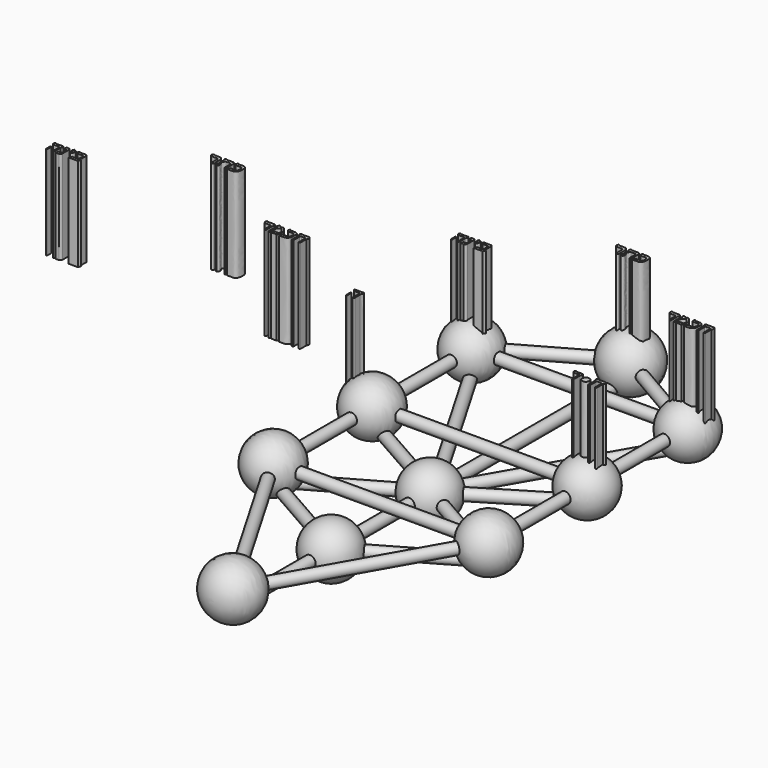
from build123d import *

# Parameters (mm, degrees)
F25_W     = 57.1091186851
F25_H     = 1.5
F25_W_2   = 52.1633550525
F38_DEPTH = 25


# Not quite as in the source:
# - ends of sketch curves that miss each other by under 0.0002 mm in the source are joined


with BuildPart() as f1:
    # F0 (on Top) → F1 (revolve)
    with BuildSketch(Plane.XY):
        with BuildLine():
            Line((-29.2246792197, -9.2726029596), (-29.2246792197, -23.7725834981))
            ThreePointArc((-29.2246792197, -23.7725834981), (-21.9628008624, -16.5225932289), (-29.2246792197, -9.2726029596))
        make_face()
    revolve(axis=Axis((-29.2246792197, -16.5225932289, 0), (0, -1, 0)))


with BuildPart() as f2:
    # F0 (on Top) → F2 (revolve)
    with BuildSketch(Plane.XY):
        with BuildLine():
            Line((28.2959174365, -23.6783408071), (28.2959174365, -9.1783614346))
            ThreePointArc((28.2959174365, -9.1783614346), (21.0581464556, -16.4283511208), (28.2959174365, -23.6783408071))
        make_face()
    revolve(axis=Axis((28.2959174365, -16.4283511208, 0), (0, -1, 0)))


with BuildPart() as f3:
    # F0 (on Top) → F3 (revolve)
    with BuildSketch(Plane.XY):
        with BuildLine():
            Line((-29.1159380303, 23.6979271757), (-29.254943913, 9.1995414743))
            ThreePointArc((-29.254943913, 9.1995414743), (-21.8528783148, 16.3784320606), (-29.1159380303, 23.6979271757))
        make_face()
    revolve(axis=Axis((-29.1854409717, 16.448734325, 0), (-0.0095872394, -0.9999540414, 0)))


with BuildPart() as f4:
    # F0 (on Top) → F4 (revolve)
    with BuildSketch(Plane.XY):
        with BuildLine():
            Line((-29.1507775773, 57.0575961277), (-29.1507775773, 42.5576208684))
            ThreePointArc((-29.1507775773, 42.5576208684), (-21.9141704929, 49.807608498), (-29.1507775773, 57.0575961277))
        make_face()
    revolve(axis=Axis((-29.1507775773, 49.807608498, 0), (0, 1, 0)))


with BuildPart() as f5:
    # F0 (on Top) → F5 (revolve)
    with BuildSketch(Plane.XY):
        with BuildLine():
            Line((-0.3091844796, -58.8778027446), (-0.3091844796, -73.3646112209))
            ThreePointArc((-0.3091844796, -73.3646112209), (7.25, -66.1212069828), (-0.3091844796, -58.8778027446))
        make_face()
    revolve(axis=Axis((-0.3091844796, -66.1212069828, 0), (0, -1, 0)))


with BuildPart() as f6:
    # F0 (on Top) → F6 (revolve)
    with BuildSketch(Plane.XY):
        with BuildLine():
            Line((35.5459174365, 16.4479395461), (21.0459174365, 16.4479395461))
            ThreePointArc((21.0459174365, 16.4479395461), (28.2959174365, 9.1979395461), (35.5459174365, 16.4479395461))
        make_face()
    revolve(axis=Axis((28.2959174365, 16.4479395461, 0), (1, 0, 0)))


with BuildPart() as f7:
    # F0 (on Top) → F7 (revolve)
    with BuildSketch(Plane.XY):
        with BuildLine():
            Line((28.5925234624, 42.4439817941), (28.5925234624, 56.9430380786))
            ThreePointArc((28.5925234624, 56.9430380786), (21.4252381199, 49.6935099363), (28.5925234624, 42.4439817941))
        make_face()
    revolve(axis=Axis((28.5925234624, 49.6935099363, 0), (0, 1, 0)))


with BuildPart() as f8:
    # F0 (on Top) → F8 (revolve)
    with BuildSketch(Plane.XY):
        with BuildLine():
            Line((0, 58.9001502285), (0, 66.3991495967))
            Line((0, 66.3991495967), (0, 73.7951572397))
            ThreePointArc((0, 73.7951572397), (-7.7135701863, 66.3476537341), (0, 58.9001502285))
        make_face()
    revolve(axis=Axis((0, 66.3476537341, 0), (0, -1, 0)))


with BuildPart() as f11:
    # F10 (on offset) → F11 (revolve)
    with BuildSketch(Plane.XY.offset(-4.1)):
        with BuildLine():
            ThreePointArc((-0.4545195449, -40.3316861829), (6.7954804551, -33.0816861829), (-0.4545195449, -25.8316861829))
            Line((-0.4545195449, -25.8316861829), (-0.4545195449, -40.3316861829))
        make_face()
    revolve(axis=Axis((-0.4545195449, -33.0816861829, -4.1), (0, -1, 0)))


with BuildPart() as f11b:
    # F10 (on offset) → F11, piece 2 (revolve)
    with BuildSketch(Plane.XY.offset(-4.1)):
        with BuildLine():
            Line((-0.4545195449, 0), (-0.4545195449, -7.25))
            ThreePointArc((-0.4545195449, -7.25), (6.7954804551, 0), (-0.4545195449, 7.25))
            Line((-0.4545195449, 7.25), (-0.4545195449, 0))
        make_face()
    revolve(axis=Axis((-0.4545195449, -33.0816861829, -4.1), (0, -1, 0)))


with BuildPart() as f13:
    # F12 (on offset) → F13 (revolve)
    with BuildSketch(Plane.XY.offset(-4.1)):
        Polygon((-26.0090909671, -16.1936523754), (-5.0356983319, -4.2643418488), (-1.3323071181, -2.1579156468), (-1.9716815625, -0.7959197113), (-5.7773049848, -2.9604938621), (-27.1052462657, -15.0914656538), align=None)
    revolve(axis=Axis((-16.4412756253, -9.025979758, -4.1), (-0.8692319911, -0.4944044353, 0)))


with BuildPart() as f14:
    # F12 (on offset) → F14 (revolve)
    with BuildSketch(Plane.XY.offset(-4.1)):
        Polygon((-1.129006822, 1.2827262948), (-0.3514380131, 0), (5.1909224811, 3.3596930733), (23.0870766217, 14.2080644789), (27.8991724979, 17.1250824535), (27.1465061848, 18.4229042555), (20.3817308309, 14.322202231), (4.3483456761, 4.603012528), align=None)
    revolve(axis=Axis((14.1389995514, 8.7838787761, -4.1), (0.8551508632, 0.5183792059, 0)))


with BuildPart() as f15:
    # F12 (on offset) → F15 (revolve)
    with BuildSketch(Plane.XY.offset(-4.1)):
        Polygon((-28.9924826053, 15.1554377692), (-25.2247012465, 13.0175819941), (-7.1870962072, 2.7829652716), (-2.8568617599, 0), (-1.9319412235, 1.525806948), (-6.4468489258, 4.0875855085), (-24.4844539652, 14.322202231), (-28.0564903249, 16.3489914295), align=None)
    revolve(axis=Axis((-15.4656514455, 9.2048938697, -4.1), (-0.8697468246, 0.4934981876, 0)))


with BuildPart() as f16:
    # F12 (on offset) → F16 (revolve)
    with BuildSketch(Plane.XY.offset(-4.1)):
        Polygon((3.2083909627, -1.937990184), (2.4637627258, -3.2401149049), (25.1154975479, -16.1936523754), (25.8601257848, -14.8915276545), align=None)
    revolve(axis=Axis((14.5342583738, -8.4147589193, -4.1), (0.8680831473, -0.4964188246, 0)))


with BuildPart() as f17:
    # F12 (on offset) → F17 (revolve)
    with BuildSketch(Plane.XY.offset(-4.1)):
        Polygon((-0.2782110823, 62.3477734625), (-1.7782110823, 62.4405108392), (-1.7782110823, 3.2196498942), (-0.2782110823, 3.2196498942), align=None)
    revolve(axis=Axis((-0.2782110823, 32.7837116783, -4.1), (0, -1, 0)))


with BuildPart() as f18:
    # F12 (on offset) → F18 (revolve)
    with BuildSketch(Plane.XY.offset(-4.1)):
        Polygon((-26.5824754433, -18.0288977431), (-27.3254525627, -19.3319652778), (-6.591141076, -31.1541606829), (-3.0596121292, -33.1677517932), (-2.3166350098, -31.8646842584), (-5.8412572049, -29.8550312084), align=None)
    revolve(axis=Axis((-16.2118663241, -23.9419644758, -4.1), (-0.8687116898, 0.4953180796, 0)))


with BuildPart() as f19:
    # F12 (on offset) → F19 (revolve)
    with BuildSketch(Plane.XY.offset(-4.1)):
        Polygon((1.202256309, -32.0779555323), (1.8714931815, -33.4234479594), (26.3763282511, -19.3291654157), (25.6284619664, -18.0288977431), align=None)
    revolve(axis=Axis((13.4153591377, -25.0534266377, -4.1), (-0.866845115, -0.4985775231, 0)))


with BuildPart() as f20:
    # F12 (on offset) → F20 (revolve)
    with BuildSketch(Plane.XY.offset(-4.1)):
        Polygon((-1.9146180712, -4.3942993507), (-1.9146180712, -26.9383080304), (-1.9146180712, -32.1800261736), (-0.4146180712, -32.1359224617), (-0.4146180712, -26.8926918507), (-0.4146180712, -4.3942993507), align=None)
    revolve(axis=Axis((-0.4146180712, -15.6434956007, -4.1), (0, -1, 0)))


with BuildPart() as f21:
    # F12 (on offset) → F21 (revolve)
    with BuildSketch(Plane.XY.offset(-4.1)):
        Polygon((-1.9687591121, -36.1691971211), (-1.9687591121, -62.2125818569), (-0.4687591121, -61.7515771825), (-0.4687591121, -37.240925887), align=None)
    revolve(axis=Axis((-0.4687591121, -49.4962515347, -4.1), (0, -1, 0)))


with BuildPart() as f23:
    # F22 (on offset) → F23 (revolve)
    with BuildSketch(Plane.XY.offset(-4.1)):
        Polygon((-28.4231418203, 49.4134207024), (-29.6505219667, 48.5401466053), (-0.8530344227, -0.9951512348), (0.4437502928, -0.2412617192), align=None)
    revolve(axis=Axis((-13.9896957638, 24.5860794916, -4.1), (-0.5025930104, 0.8645231437, 0)))


with BuildPart() as f24:
    # F22 (on offset) → F24 (revolve)
    with BuildSketch(Plane.XY.offset(-4.1)):
        Polygon((1.2984194251, 0.5149673192), (27.8307806202, 46.3830051455), (26.6649877391, 47.3633549421), (0, 1.266037886), align=None)
    revolve(axis=Axis((13.3324938695, 24.314696414, -4.1), (0.5007137112, 0.8656129501, 0)))


with BuildPart() as f26:
    # F25 (on Top) → F26 (revolve)
    with BuildSketch(Plane.XY):
        Polygon((-2.2483841008, 67.0031690276), (-27.4323771774, 52.753087862), (-26.6936765174, 51.4475912764), (-1.5096834408, 65.697672442), align=None)
    revolve(axis=Axis((-14.1016799791, 58.5726318592, 0), (0.8703310571, 0.4924671066, 0)))


with BuildPart() as f27:
    # F25 (on Top) → F27 (revolve)
    with BuildSketch(Plane.XY):
        Polygon((24.2450092439, 51.9837853236), (24.9992646277, 53.2803572714), (4.7837163632, 65.0403572773), (3.7131184762, 63.9278113964), align=None)
    revolve(axis=Axis((13.9790638601, 57.95579836, 0), (-0.8643812986, 0.5028369225, 0)))


with BuildPart() as f28:
    # F25 (on Top) → F28 (revolve)
    with BuildSketch(Plane.XY):
        with Locations((-0.4721774086, 49.1002261341)):
            Rectangle(F25_W, F25_H)
    revolve(axis=Axis((-0.4721774086, 49.8502261341, 0), (-1, 0, 0)))


with BuildPart() as f29:
    # F25 (on Top) → F29 (revolve)
    with BuildSketch(Plane.XY):
        with Locations((-0.4721774086, 16.0002366511)):
            Rectangle(F25_W, F25_H)
    revolve(axis=Axis((-0.4721774086, 16.7502366511, 0), (1, 0, 0)))


with BuildPart() as f30:
    # F25 (on Top) → F30 (revolve)
    with BuildSketch(Plane.XY):
        with Locations((-0.9874179959, -17.2000393569)):
            Rectangle(F25_W_2, F25_H)
    revolve(axis=Axis((-0.9874179959, -16.4500393569, 0), (1, 0, 0)))


with BuildPart() as f31:
    # F25 (on Top) → F31 (revolve)
    with BuildSketch(Plane.XY):
        Polygon((-30.5267367512, 47.590128925), (-30.5267367512, 16.7502366511), (-29.0267367512, 16.7502366511), (-29.0267367512, 47.590128925), (-29.0267367512, 48.3502261341), (-29.0267367512, 49.8502261341), (-29.0267367512, 55.475987494), (-30.5267367512, 55.475987494), align=None)
    revolve(axis=Axis((-29.0267367512, 15.1780908165, 0), (0, -1, 0)))


with BuildPart() as f32:
    # F25 (on Top) → F32 (revolve)
    with BuildSketch(Plane.XY):
        Polygon((-30.5267367512, 15.2502366511), (-30.5267367512, -17.0896556228), (-29.0267367512, -17.233947292), (-29.0267367512, -16.4500393569), (-29.0267367512, 15.2502366511), align=None)
    revolve(axis=Axis((-29.0267367512, 15.1780908165, 0), (0, -1, 0)))


with BuildPart() as f33:
    # F25 (on Top) → F33 (revolve)
    with BuildSketch(Plane.XY):
        Polygon((28.0823819339, 47.590128925), (28.0823819339, 16.7502366511), (29.5823819339, 16.7502366511), (29.5823819339, 47.590128925), (29.5823819339, 53.9458170533), (28.0823819339, 53.9458170533), (28.0823819339, 49.8502261341), (28.0823819339, 48.3502261341), align=None)
    revolve(axis=Axis((28.0823819339, 15.1531686244, 0), (0, -1, 0)))


with BuildPart() as f34:
    # F25 (on Top) → F34 (revolve)
    with BuildSketch(Plane.XY):
        Polygon((29.5823819339, 15.2502366511), (28.0823819339, 15.2502366511), (28.0823819339, -17.2837916762), (29.5823819339, -17.0896556228), align=None)
    revolve(axis=Axis((28.0823819339, 15.1531686244, 0), (0, -1, 0)))


with BuildPart() as f35:
    # F25 (on Top) → F35 (revolve)
    with BuildSketch(Plane.XY):
        Polygon((-28.1386089989, -18.5248188859), (-29.4354074421, -19.2786847874), (-3.025480399, -64.7089824118), (-2.2920486471, -62.9860143837), align=None)
    revolve(axis=Axis((-15.215328823, -40.7554166348, 0), (0.5025772677, -0.8645322955, 0)))


with BuildPart() as f36:
    # F25 (on Top) → F36 (revolve)
    with BuildSketch(Plane.XY):
        Polygon((25.1791188454, -18.5248188859), (0, -62.7821208306), (1.3037680308, -63.5238680396), (26.4828868762, -19.2665660948), align=None)
    revolve(axis=Axis((13.8933274535, -41.3952170672, 0), (-0.4944981393, -0.8691786872, 0)))


with BuildPart() as f38:
    # F37 (on Top) → F38 (new body)
    with BuildSketch(Plane.XY):
        with BuildLine():
            ThreePointArc((-3.0653644353, 67.1784728765), (-2.8025297919, 67.0878512001), (-2.6513966732, 66.8544992805))
            Line((-2.6513966732, 66.8544992805), (-2.6513966732, 64.9466440082))
            ThreePointArc((-2.6513966732, 64.9466440082), (-2.336421283, 64.6316686179), (-2.0214458928, 64.9466440082))
            Line((-2.0214458928, 64.9466440082), (-2.0214458928, 67.0884773135))
            ThreePointArc((-2.0214458928, 67.0884773135), (-2.2850278392, 67.7248260114), (-2.921375446, 67.9884105921))
            Line((-2.921375446, 67.9884105921), (-4.2892689817, 67.9884105921))
            Line((-4.2892689817, 67.9884105921), (-4.5412490144, 68.204395473))
            ThreePointArc((-4.5412490144, 68.204395473), (-4.849471547, 67.6038104444), (-4.3252659962, 67.1784728765))
            Line((-4.3252659962, 67.1784728765), (-3.0653644353, 67.1784728765))
        make_face()
    extrude(amount=F38_DEPTH)


with BuildPart() as f38b:
    # F37 (on Top) → F38, piece 2 (new body)
    with BuildSketch(Plane.XY):
        with BuildLine():
            Line((0.8917081286, 67.944958806), (-0.9845615132, 67.944958806))
            Line((-0.9845615132, 67.944958806), (-1.2270726729, 68.212993443))
            ThreePointArc((-1.2270726729, 68.212993443), (-1.4705783197, 67.695205533), (-1.1760175694, 67.2046616673))
            Line((-1.1760175694, 67.2046616673), (-0.9845615132, 67.2046616673))
            ThreePointArc((-0.9845615132, 67.2046616673), (-1.3399701386, 66.7916285787), (-1.4562645229, 66.2592872977))
            add(Edge.make_bspline(
                [(-1.4562645229, 66.2592872977), (-1.298919821, 65.9481865812), (-1.1415751191, 65.6370858647), (-1.0664021829, 65.6477361917)],
                knots=[0, 0, 0, 0, 0.6206613071, 0.6206613071, 0.6206613071, 0.6206613071], degree=3))
            Line((-1.0664021829, 65.6477361917), (-1.0664021829, 65.4260516167))
            ThreePointArc((-1.0664021829, 65.4260516167), (-1.524823322, 65.0552995503), (-1.0664021829, 64.6845474839))
            add(Edge.make_bspline(
                [(-1.0664021829, 64.6845474839), (-0.9299616228, 64.7280319877), (-0.6148415588, 64.8284628244), (-0.6660040244, 65.6043238446), (-0.9807793236, 66.1163927423), (-1.1103381456, 66.31969189), (-0.936011435, 66.6878671178), (-0.6815481934, 67.0875361163), (-0.549417983, 67.1355030055), (-0.4995394265, 67.1536102891)],
                knots=[0, 0, 0, 0, 0.143013218, 0.3303001276, 0.5069381179, 0.6093778874, 0.749431031, 0.9054113483, 1, 1, 1, 1], degree=3))
            Line((-0.4995394265, 67.1536102891), (0.5726146046, 67.1536102891))
            ThreePointArc((0.5726146046, 67.1536102891), (0.7713780161, 67.076519404), (0.8661806351, 66.8855682015))
            Line((0.8661806351, 66.8855682015), (0.8661806351, 64.8816600442))
            add(Edge.make_bspline(
                [(0.8661806351, 64.8816600442), (0.9637554989, 64.6672288611), (1.107026649, 64.7118448217), (1.2345502619, 64.6769031882), (1.3129115105, 64.8178458214)],
                knots=[0, 0, 0, 0, 0.5338591793, 1, 1, 1, 1], degree=3))
            Line((1.3129115105, 64.8178458214), (1.3129115105, 67.3833563924))
            ThreePointArc((1.3129115105, 67.3833563924), (1.1959105012, 67.7343583724), (0.8917081286, 67.944958806))
        make_face()
    extrude(amount=F38_DEPTH)


with BuildPart() as f38c:
    # F37 (on Top) → F38, piece 3 (new body)
    with BuildSketch(Plane.XY):
        with BuildLine():
            Line((2.165451413, 67.9095983505), (1.9481471973, 68.1726559997))
            add(Edge.make_bspline(
                [(3.2571300399, 65.4171183705), (3.3416971608, 65.403090998), (3.5378047086, 65.3705621192), (3.9276989444, 65.7256632725), (3.8849798648, 66.7011834402), (3.6673793109, 67.1280083292), (3.2415806497, 67.1582747194), (2.4631242872, 67.1807870502), (1.941314711, 67.1067176355), (1.6369969691, 67.6034814899), (1.8386144265, 67.9722921386), (1.9481471973, 68.1726559997)],
                knots=[0, 0, 0, 0, 0.0782388208, 0.1814324895, 0.3324909078, 0.4331194472, 0.5284864943, 0.6667138036, 0.7749860041, 0.8777565855, 1, 1, 1, 1], degree=3))
            Line((3.2571300399, 65.4171183705), (1.9603001419, 65.4171183705))
            Line((1.9603001419, 65.4171183705), (1.6954155872, 64.7052377462))
            add(Edge.make_bspline(
                [(2.165451413, 67.9095983505), (2.6628579125, 67.9472770571), (3.4977054742, 68.0105364449), (4.1163767034, 67.6688910219), (4.3949006426, 67.2671741331), (4.4605693583, 65.6218115304), (3.8565194054, 64.7724261534), (3.3259863253, 64.6584547091), (2.3300345056, 64.6997243166), (1.6954155872, 64.7052377462)],
                knots=[0, 0, 0, 0, 0.1703298867, 0.2852071147, 0.3832734237, 0.5680244438, 0.7110133222, 0.8119163737, 1, 1, 1, 1], degree=3))
        make_face()
    extrude(amount=F38_DEPTH)


with BuildPart() as f38d:
    # F37 (on Top) → F38, piece 4 (new body)
    with BuildSketch(Plane.XY):
        with BuildLine():
            Line((25.094807148, 51.4051318169), (23.204844445, 51.4051318169))
            Line((23.204844445, 51.4051318169), (23.0134855956, 51.5683069825))
            ThreePointArc((23.0134855956, 51.5683069825), (22.8077149881, 50.9523500645), (23.3320537955, 50.5691878498))
            Line((23.3320537955, 50.5691878498), (24.4769342244, 50.5691878498))
            ThreePointArc((24.4769342244, 50.5691878498), (24.7026346594, 50.4641835546), (24.7676968575, 50.2239055932))
            Line((24.7676968575, 50.2239055932), (24.7676968575, 48.4611541033))
            ThreePointArc((24.7676968575, 48.4611541033), (24.9820259039, 48.1801464248), (25.2428222448, 48.4186574814))
            Line((25.2428222448, 48.4186574814), (25.2428222448, 50.1814074814))
            add(Edge.make_bspline(
                [(25.094807148, 51.4051318169), (25.2333902782, 51.3246485973), (25.498607664, 51.170621559), (25.4409015348, 50.743700745), (25.2031096306, 50.4888201492), (25.2298890891, 50.2815221669), (25.2428222448, 50.1814074814)],
                knots=[0, 0, 0, 0, 0.2771912277, 0.5304825536, 0.7732462663, 1, 1, 1, 1], degree=3))
        make_face()
    extrude(amount=F38_DEPTH)


with BuildPart() as f38e:
    # F37 (on Top) → F38, piece 5 (new body)
    with BuildSketch(Plane.XY):
        with BuildLine():
            add(Edge.make_bspline(
                [(25.9900391102, 49.950491637), (26.1744233596, 50.3653591183), (26.598168419, 50.5068944279), (26.3755768751, 50.5890751322), (26.093079649, 50.7040706647), (25.9207844085, 51.1238085009), (26.1227499571, 51.5132743631), (26.319645307, 51.6342521033), (26.2693582845, 51.3990660305), (26.6722261078, 51.3917805678), (26.9070038169, 51.2977939427), (26.9182347005, 50.8240999202), (27.0431924073, 50.8574435474), (27.2164904687, 50.7971375085), (26.9361725288, 51.475505852), (27.5748879862, 51.3555270066), (27.7282123667, 51.2735150805), (28.2909398678, 50.4875646707), (28.5934648423, 50.0452560881), (28.610871723, 48.3027908308), (28.2914711547, 48.2310240701), (28.1424051351, 48.1103625657)],
                knots=[0, 0, 0, 0, 0.0756054344, 0.1035718875, 0.1515665723, 0.2072022695, 0.2643515876, 0.2965819361, 0.3273272823, 0.3780622313, 0.4212250999, 0.475223405, 0.5013702445, 0.5272235095, 0.5862652195, 0.6424805002, 0.6829170985, 0.7638694334, 0.8341339003, 0.9411916895, 1, 1, 1, 1], degree=3))
            Line((25.9900391102, 49.950491637), (25.9900391102, 48.1999628246))
            ThreePointArc((25.9900391102, 48.1999628246), (26.2316696606, 48.0641239759), (26.4090355486, 48.2771471143))
            Line((26.4090355486, 48.2771471143), (26.4090355486, 49.7987680137))
            add(Edge.make_bspline(
                [(27.9637351632, 48.8615371287), (28.0519759366, 48.8737126093), (28.2886236947, 48.9063147191), (28.2877700432, 49.7519870139), (27.67774579, 50.5432709715), (27.0828288789, 50.7396636964), (26.5413504094, 50.1185283065), (26.4090355486, 49.7987680137)],
                knots=[0, 0, 0, 0, 0.1226385123, 0.3294930755, 0.573496868, 0.7473063095, 1, 1, 1, 1], degree=3))
            Line((27.9637351632, 48.8615371287), (27.0265042782, 48.8615371287))
            Line((27.0265042782, 48.8615371287), (26.7530990965, 48.1103625657))
            Line((26.7530990965, 48.1103625657), (28.1424051351, 48.1103625657))
        make_face()
    extrude(amount=F38_DEPTH)


with BuildPart() as f38f:
    # F37 (on Top) → F38, piece 6 (new body)
    with BuildSketch(Plane.XY):
        with BuildLine():
            add(Edge.make_bspline(
                [(29.3763037771, 51.3518042862), (29.9669969827, 51.2805134058), (30.5416331701, 51.3393142133), (31.048751742, 51.2305894269), (31.4975495224, 50.856803983), (31.4391660861, 50.2012074651), (31.5269753407, 49.1707961225), (31.2381665172, 48.5625305376), (30.6566903466, 47.9457524877), (29.5370743399, 48.0184536125), (28.8708265871, 48.0421744287)],
                knots=[0, 0, 0, 0, 0.1516832683, 0.2445742042, 0.3415191393, 0.4507555344, 0.5898563647, 0.7003176737, 0.8172659573, 1, 1, 1, 1], degree=3))
            add(Edge.make_bspline(
                [(29.1409362108, 48.8290153444), (29.6073883642, 48.809220721), (30.3655227478, 48.776535883), (30.9561657401, 48.9532139835), (31.0585535543, 49.5080904147), (31.0969904137, 50.2122581004), (30.793647648, 50.6179884493), (30.5427362406, 50.6818232794), (29.9119888446, 50.607220348), (28.9749989681, 50.7020638732), (28.8943312929, 51.1566845874), (29.1451182919, 51.8788034456), (29.2603092689, 51.3048671151), (29.3763037771, 51.3518042862)],
                knots=[0, 0, 0, 0, 0.1374282589, 0.2251579074, 0.3118855155, 0.4151962191, 0.4970093193, 0.5550611878, 0.6536030387, 0.766823688, 0.8461414177, 0.9276947987, 1, 1, 1, 1], degree=3))
            Line((29.1409362108, 48.8290153444), (28.8708265871, 48.0421744287))
        make_face()
    extrude(amount=F38_DEPTH)


with BuildPart() as f38g:
    # F37 (on Top) → F38, piece 7 (new body)
    with BuildSketch(Plane.XY):
        with BuildLine():
            add(Edge.make_bspline(
                [(32.1654975414, 50.311550498), (32.1540758014, 50.5299642682), (32.6390919211, 50.6330340488), (32.397514, 50.6551574719), (32.3272198439, 50.6541989744)],
                knots=[0, 0, 0, 0, 0.6308602652, 1, 1, 1, 1], degree=3))
            Line((32.1654975414, 50.311550498), (32.1654975414, 48.2255779207))
            ThreePointArc((32.1654975414, 48.2255779207), (32.3943684426, 48.0907731131), (32.6172970235, 48.2351928949))
            Line((32.6172970235, 48.2351928949), (32.6172970235, 50.2923242748))
            add(Edge.make_bspline(
                [(32.6172970235, 50.2923242748), (32.605689019, 50.5695864558), (32.7056571841, 50.6047904491), (32.9169668257, 50.5925826728)],
                knots=[0, 0, 0, 0, 0.4242135028, 0.4242135028, 0.4242135028, 0.4242135028], degree=3))
            Line((32.9169668257, 50.5925826728), (33.6827635765, 50.5925826728))
            ThreePointArc((33.6827635765, 50.5925826728), (33.9581384614, 50.4578494471), (34.0207591653, 50.1577444375))
            Line((34.0207591653, 50.1577444375), (34.0207591653, 48.2351928949))
            ThreePointArc((34.0207591653, 48.2351928949), (34.2597436555, 48.1282020934), (34.4210900366, 48.334425185))
            Line((34.4210900366, 48.334425185), (34.4210900366, 50.3110513091))
            add(Edge.make_bspline(
                [(34.4210900366, 50.3110513091), (34.4723193627, 50.3874964826), (34.5758126022, 50.5419306562), (34.6811156751, 50.8223443744), (34.680047203, 50.9489657432), (34.6795804799, 51.0042756796)],
                knots=[0, 0, 0, 0, 0.3556858258, 0.7185548037, 1, 1, 1, 1], degree=3))
            ThreePointArc((34.6795804799, 51.0042756796), (34.4830908157, 51.2884676727), (34.1553390026, 51.397792995))
            Line((34.1553390026, 51.397792995), (32.3962047696, 51.397792995))
            Line((32.3962047696, 51.397792995), (32.2428362886, 51.3939732407))
            Line((32.2428362886, 51.3939732407), (32.2215929627, 51.5696294606))
            ThreePointArc((32.2215929627, 51.5696294606), (31.9202023544, 51.0710444086), (32.3272198439, 50.6541989744))
        make_face()
    extrude(amount=F38_DEPTH)


with BuildPart() as f38h:
    # F37 (on Top) → F38, piece 8 (new body)
    with BuildSketch(Plane.XY):
        with BuildLine():
            ThreePointArc((-33.1885628402, 49.69278723), (-33.3940379587, 49.7795182839), (-33.5302054882, 49.602881074))
            Line((-33.5302054882, 49.602881074), (-33.5302054882, 48.3441911638))
            ThreePointArc((-33.5302054882, 48.3441911638), (-33.3593841642, 48.1733698398), (-33.1885628402, 48.3441911638))
            Line((-33.1885628402, 48.3441911638), (-33.1885628402, 49.69278723))
        make_face()
    extrude(amount=F38_DEPTH)


with BuildPart() as f38i:
    # F37 (on Top) → F38, piece 9 (new body)
    with BuildSketch(Plane.XY):
        with BuildLine():
            ThreePointArc((-32.1466326714, 50.6696887314), (-31.8911760421, 50.6312510432), (-31.7733027041, 50.401378423))
            Line((-31.7733027041, 50.401378423), (-31.7733027041, 48.3948066831))
            ThreePointArc((-31.7733027041, 48.3948066831), (-31.5895192325, 48.2110232115), (-31.4057357609, 48.3948066831))
            Line((-31.4057357609, 48.3948066831), (-31.4057357609, 50.3690131009))
            add(Edge.make_bspline(
                [(-31.4057357609, 50.3690131009), (-31.4095837692, 50.4189937627), (-31.4295884678, 50.5171076828), (-31.258597526, 50.6366704829), (-31.0965974663, 51.3214918455), (-31.4006780135, 51.3895071545), (-31.5616987646, 51.3741709292)],
                knots=[0, 0, 0, 0, 0.1663027448, 0.3682274229, 0.7199979536, 1, 1, 1, 1], degree=3))
            Line((-31.5616987646, 51.3741709292), (-33.4339700639, 51.3741709292))
            Line((-33.4339700639, 51.3741709292), (-33.5380919278, 51.5973269939))
            ThreePointArc((-33.5380919278, 51.5973269939), (-33.8109817037, 51.1335078627), (-33.5380919278, 50.6696887314))
            Line((-33.5380919278, 50.6696887314), (-32.1466326714, 50.6696887314))
        make_face()
    extrude(amount=F38_DEPTH)


with BuildPart() as f38j:
    # F37 (on Top) → F38, piece 10 (new body)
    with BuildSketch(Plane.XY):
        with BuildLine():
            Line((-30.3256213665, 50.6855100393), (-29.9883969128, 50.6114475429))
            add(Edge.make_bspline(
                [(-29.9883969128, 50.6114475429), (-29.9129808499, 50.5243950231), (-29.7441789029, 50.3739905454), (-29.7908920969, 49.3009830151), (-29.8124247461, 48.858817547), (-30.3178911482, 48.8691939216), (-30.6207705289, 48.884216696)],
                knots=[0, 0, 0, 0, 0.1869413092, 0.5223132524, 0.7192998021, 1, 1, 1, 1], degree=3))
            Line((-30.6207705289, 48.884216696), (-30.8993477374, 48.1262244284))
            Line((-30.8993477374, 48.1262244284), (-30.0088264048, 48.1262244284))
            add(Edge.make_bspline(
                [(-30.0088264048, 48.1262244284), (-29.9267658275, 48.1566826516), (-29.7533640682, 48.2205004754), (-29.550597883, 48.4886712737), (-29.5136149565, 48.6174046687), (-29.5017529279, 48.6735254526)],
                knots=[0, 0, 0, 0, 0.3416646173, 0.7156481816, 1, 1, 1, 1], degree=3))
            Line((-29.5017529279, 48.6735254526), (-29.5017529279, 50.9821027517))
            ThreePointArc((-29.5017529279, 50.9821027517), (-29.6216762446, 51.2549916443), (-29.9038011581, 51.3511970639))
            Line((-29.9038011581, 51.3511970639), (-30.2629191428, 51.4086149633))
            Line((-30.2629191428, 51.4086149633), (-30.3377602249, 51.5208765864))
            ThreePointArc((-30.3377602249, 51.5208765864), (-30.5743034624, 51.0996678655), (-30.3256213665, 50.6855100393))
        make_face()
    extrude(amount=F38_DEPTH)


with BuildPart() as f38k:
    # F37 (on Top) → F38, piece 11 (new body)
    with BuildSketch(Plane.XY):
        with BuildLine():
            Line((-28.3746067435, 51.3340570033), (-28.5574216396, 51.414038986))
            add(Edge.make_bspline(
                [(-28.1024370342, 51.3340570033), (-28.0513590215, 51.3201760449), (-27.9020187049, 51.308858898), (-27.9042867012, 51.148640236), (-27.7667519085, 50.5179182547), (-28.1095169748, 50.2042261439), (-28.2853246315, 49.9044469684), (-28.5122822086, 49.873588393), (-28.4279102681, 50.1060425542), (-28.0612465573, 50.4354569269), (-28.0954403381, 50.5835884211), (-28.1479497897, 50.6958640353), (-28.3357909045, 50.7423431044), (-28.6536959234, 50.6278964805), (-28.8461082751, 50.8619518654), (-28.8748633654, 51.1925415324), (-28.7614154579, 51.4728880694), (-28.592347498, 51.6814073048), (-28.6615811058, 51.374027441), (-28.5859130931, 51.4030943482), (-28.5574216396, 51.414038986)],
                knots=[0, 0, 0, 0, 0.0480600535, 0.0899223282, 0.1792705215, 0.2568386321, 0.3243074746, 0.3671550691, 0.4151636097, 0.4964581018, 0.5375246526, 0.5753688461, 0.6237252983, 0.6878848584, 0.74557128, 0.8109553318, 0.8778038857, 0.9205228557, 0.9698196046, 1, 1, 1, 1], degree=3))
            Line((-28.1024370342, 51.3340570033), (-28.3746067435, 51.3340570033))
        make_face()
    extrude(amount=F38_DEPTH)


with BuildPart() as f38l:
    # F37 (on Top) → F38, piece 12 (new body)
    with BuildSketch(Plane.XY):
        with BuildLine():
            ThreePointArc((-25.7367603481, 50.6524220109), (-25.5275964164, 50.5942022382), (-25.3785923123, 50.4362881184))
            Line((-25.3785923123, 50.4362881184), (-25.3785923123, 49.0150637925))
            ThreePointArc((-25.3785923123, 49.0150637925), (-25.4295327596, 48.9032951387), (-25.5473079183, 48.8684214652))
            Line((-25.5473079183, 48.8684214652), (-27.0456110919, 48.8684214652))
            Line((-27.0456110919, 48.8684214652), (-27.3683071136, 48.1244288385))
            Line((-27.3683071136, 48.1244288385), (-24.9238014221, 48.1244288385))
            Line((-24.9238014221, 48.1244288385), (-24.6324073761, 48.8737225533))
            Line((-24.6324073761, 48.8737225533), (-24.933276698, 48.8737225533))
            Line((-24.933276698, 48.8737225533), (-24.933276698, 50.9574003518))
            ThreePointArc((-24.933276698, 50.9574003518), (-25.0649270069, 51.265540991), (-25.3785923123, 51.3834245503))
            Line((-25.3785923123, 51.3834245503), (-27.0716361701, 51.3834245503))
            Line((-27.0716361701, 51.3834245503), (-27.0716361701, 51.5953116119))
            ThreePointArc((-27.0716361701, 51.5953116119), (-27.3772515988, 51.1238668114), (-27.0716361701, 50.6524220109))
            Line((-27.0716361701, 50.6524220109), (-25.7367603481, 50.6524220109))
        make_face()
    extrude(amount=F38_DEPTH)


with BuildPart() as f38m:
    # F37 (on Top) → F38, piece 13 (new body)
    with BuildSketch(Plane.XY):
        with BuildLine():
            ThreePointArc((-94.5650778354, 46.2948548295), (-94.302243192, 46.204233153), (-94.1511100732, 45.9708812334))
            Line((-94.1511100732, 45.9708812334), (-94.1511100732, 44.0630259611))
            ThreePointArc((-94.1511100732, 44.0630259611), (-93.836134683, 43.7480505709), (-93.5211592928, 44.0630259611))
            Line((-93.5211592928, 44.0630259611), (-93.5211592928, 46.2048592664))
            ThreePointArc((-93.5211592928, 46.2048592664), (-93.7847412393, 46.8412079643), (-94.4210888461, 47.104792545))
            Line((-94.4210888461, 47.104792545), (-95.7889823817, 47.104792545))
            Line((-95.7889823817, 47.104792545), (-96.0409624145, 47.3207774259))
            ThreePointArc((-96.0409624145, 47.3207774259), (-96.3491849471, 46.7201923973), (-95.8249793962, 46.2948548295))
            Line((-95.8249793962, 46.2948548295), (-94.5650778354, 46.2948548295))
        make_face()
    extrude(amount=F38_DEPTH)


with BuildPart() as f38n:
    # F37 (on Top) → F38, piece 14 (new body)
    with BuildSketch(Plane.XY):
        with BuildLine():
            Line((-90.6080052714, 47.0613407589), (-92.4842749132, 47.0613407589))
            Line((-92.4842749132, 47.0613407589), (-92.726786073, 47.3293753959))
            ThreePointArc((-92.726786073, 47.3293753959), (-92.9702917197, 46.8115874859), (-92.6757309694, 46.3210436203))
            Line((-92.6757309694, 46.3210436203), (-92.4842749132, 46.3210436203))
            ThreePointArc((-92.4842749132, 46.3210436203), (-92.8396835386, 45.9080105317), (-92.9559779229, 45.3756692506))
            add(Edge.make_bspline(
                [(-92.9559779229, 45.3756692506), (-92.7986332211, 45.0645685341), (-92.6412885192, 44.7534678176), (-92.566115583, 44.7641181447)],
                knots=[0, 0, 0, 0, 0.6206613071, 0.6206613071, 0.6206613071, 0.6206613071], degree=3))
            Line((-92.566115583, 44.7641181447), (-92.566115583, 44.5424335696))
            ThreePointArc((-92.566115583, 44.5424335696), (-93.0245367221, 44.1716815032), (-92.566115583, 43.8009294368))
            add(Edge.make_bspline(
                [(-92.566115583, 43.8009294368), (-92.4296750229, 43.8444139406), (-92.1145549589, 43.9448447773), (-92.1657174245, 44.7207057975), (-92.4804927237, 45.2327746952), (-92.6100515457, 45.4360738429), (-92.4357248351, 45.8042490707), (-92.1812615935, 46.2039180692), (-92.049131383, 46.2518849584), (-91.9992528266, 46.269992242)],
                knots=[0, 0, 0, 0, 0.143013218, 0.3303001276, 0.5069381179, 0.6093778874, 0.749431031, 0.9054113483, 1, 1, 1, 1], degree=3))
            Line((-91.9992528266, 46.269992242), (-90.9270987955, 46.269992242))
            ThreePointArc((-90.9270987955, 46.269992242), (-90.728335384, 46.1929013569), (-90.633532765, 46.0019501544))
            Line((-90.633532765, 46.0019501544), (-90.633532765, 43.9980419971))
            add(Edge.make_bspline(
                [(-90.633532765, 43.9980419971), (-90.5359579012, 43.783610814), (-90.392686751, 43.8282267746), (-90.2651631382, 43.7932851411), (-90.1868018896, 43.9342277743)],
                knots=[0, 0, 0, 0, 0.5338591793, 1, 1, 1, 1], degree=3))
            Line((-90.1868018896, 43.9342277743), (-90.1868018896, 46.4997383453))
            ThreePointArc((-90.1868018896, 46.4997383453), (-90.3038028988, 46.8507403253), (-90.6080052714, 47.0613407589))
        make_face()
    extrude(amount=F38_DEPTH)


with BuildPart() as f38o:
    # F37 (on Top) → F38, piece 15 (new body)
    with BuildSketch(Plane.XY):
        with BuildLine():
            Line((-89.334261987, 47.0259803034), (-89.5515662028, 47.2890379526))
            add(Edge.make_bspline(
                [(-88.2425833602, 44.5335003234), (-88.1580162393, 44.5194729509), (-87.9619086915, 44.4869440721), (-87.5720144556, 44.8420452255), (-87.6147335353, 45.8175653931), (-87.8323340892, 46.2443902821), (-88.2581327503, 46.2746566723), (-89.0365891129, 46.2971690031), (-89.5583986891, 46.2230995885), (-89.862716431, 46.7198634428), (-89.6610989735, 47.0886740915), (-89.5515662028, 47.2890379526)],
                knots=[0, 0, 0, 0, 0.0782388208, 0.1814324895, 0.3324909078, 0.4331194472, 0.5284864943, 0.6667138036, 0.7749860041, 0.8777565855, 1, 1, 1, 1], degree=3))
            Line((-88.2425833602, 44.5335003234), (-89.5394132581, 44.5335003234))
            Line((-89.5394132581, 44.5335003234), (-89.8042978129, 43.8216196991))
            add(Edge.make_bspline(
                [(-89.334261987, 47.0259803034), (-88.8368554876, 47.06365901), (-88.0020079259, 47.1269183978), (-87.3833366966, 46.7852729748), (-87.1048127575, 46.383556086), (-87.0391440417, 44.7381934833), (-87.6431939947, 43.8888081063), (-88.1737270747, 43.774836662), (-89.1696788945, 43.8161062695), (-89.8042978129, 43.8216196991)],
                knots=[0, 0, 0, 0, 0.1703298867, 0.2852071147, 0.3832734237, 0.5680244438, 0.7110133222, 0.8119163737, 1, 1, 1, 1], degree=3))
        make_face()
    extrude(amount=F38_DEPTH)


with BuildPart() as f38p:
    # F37 (on Top) → F38, piece 16 (new body)
    with BuildSketch(Plane.XY):
        with BuildLine():
            Line((-66.4049062521, 30.5215137698), (-68.2948689551, 30.5215137698))
            Line((-68.2948689551, 30.5215137698), (-68.4862278045, 30.6846889354))
            ThreePointArc((-68.4862278045, 30.6846889354), (-68.6919984119, 30.0687320174), (-68.1676596046, 29.6855698027))
            Line((-68.1676596046, 29.6855698027), (-67.0227791757, 29.6855698027))
            ThreePointArc((-67.0227791757, 29.6855698027), (-66.7970787406, 29.5805655075), (-66.7320165426, 29.3402875461))
            Line((-66.7320165426, 29.3402875461), (-66.7320165426, 27.5775360562))
            ThreePointArc((-66.7320165426, 27.5775360562), (-66.5176874961, 27.2965283777), (-66.2568911553, 27.5350394343))
            Line((-66.2568911553, 27.5350394343), (-66.2568911553, 29.2977894343))
            add(Edge.make_bspline(
                [(-66.4049062521, 30.5215137698), (-66.2663231219, 30.4410305502), (-66.0011057361, 30.2870035119), (-66.0588118653, 29.8600826979), (-66.2966037694, 29.6052021021), (-66.2698243109, 29.3979041198), (-66.2568911553, 29.2977894343)],
                knots=[0, 0, 0, 0, 0.2771912277, 0.5304825536, 0.7732462663, 1, 1, 1, 1], degree=3))
        make_face()
    extrude(amount=F38_DEPTH)


with BuildPart() as f38q:
    # F37 (on Top) → F38, piece 17 (new body)
    with BuildSketch(Plane.XY):
        with BuildLine():
            add(Edge.make_bspline(
                [(-65.5096742899, 29.0668735899), (-65.3252900405, 29.4817410712), (-64.901544981, 29.6232763808), (-65.124136525, 29.7054570851), (-65.4066337511, 29.8204526176), (-65.5789289916, 30.2401904538), (-65.376963443, 30.629656316), (-65.180068093, 30.7506340562), (-65.2303551155, 30.5154479834), (-64.8274872923, 30.5081625207), (-64.5927095832, 30.4141758956), (-64.5814786996, 29.9404818731), (-64.4565209928, 29.9738255003), (-64.2832229314, 29.9135194615), (-64.5635408713, 30.5918878049), (-63.9248254138, 30.4719089595), (-63.7715010334, 30.3898970334), (-63.2087735323, 29.6039466236), (-62.9062485578, 29.161638041), (-62.8888416771, 27.4191727837), (-63.2082422454, 27.347406023), (-63.3573082649, 27.2267445186)],
                knots=[0, 0, 0, 0, 0.0756054344, 0.1035718875, 0.1515665723, 0.2072022695, 0.2643515876, 0.2965819361, 0.3273272823, 0.3780622313, 0.4212250999, 0.475223405, 0.5013702445, 0.5272235095, 0.5862652195, 0.6424805002, 0.6829170985, 0.7638694334, 0.8341339003, 0.9411916895, 1, 1, 1, 1], degree=3))
            Line((-65.5096742899, 29.0668735899), (-65.5096742899, 27.3163447775))
            ThreePointArc((-65.5096742899, 27.3163447775), (-65.2680437395, 27.1805059288), (-65.0906778515, 27.3935290672))
            Line((-65.0906778515, 27.3935290672), (-65.0906778515, 28.9151499666))
            add(Edge.make_bspline(
                [(-63.5359782368, 27.9779190816), (-63.4477374634, 27.9900945622), (-63.2110897053, 28.022696672), (-63.2119433568, 28.8683689668), (-63.82196761, 29.6596529244), (-64.4168845212, 29.8560456493), (-64.9583629907, 29.2349102594), (-65.0906778515, 28.9151499666)],
                knots=[0, 0, 0, 0, 0.1226385123, 0.3294930755, 0.573496868, 0.7473063095, 1, 1, 1, 1], degree=3))
            Line((-63.5359782368, 27.9779190816), (-64.4732091219, 27.9779190816))
            Line((-64.4732091219, 27.9779190816), (-64.7466143035, 27.2267445186))
            Line((-64.7466143035, 27.2267445186), (-63.3573082649, 27.2267445186))
        make_face()
    extrude(amount=F38_DEPTH)


with BuildPart() as f38r:
    # F37 (on Top) → F38, piece 18 (new body)
    with BuildSketch(Plane.XY):
        with BuildLine():
            add(Edge.make_bspline(
                [(-62.123409623, 30.4681862391), (-61.5327164174, 30.3968953587), (-60.95808023, 30.4556961662), (-60.4509616581, 30.3469713799), (-60.0021638777, 29.9731859359), (-60.060547314, 29.317589418), (-59.9727380594, 28.2871780754), (-60.2615468829, 27.6789124905), (-60.8430230535, 27.0621344406), (-61.9626390602, 27.1348355654), (-62.628886813, 27.1585563816)],
                knots=[0, 0, 0, 0, 0.1516832683, 0.2445742042, 0.3415191393, 0.4507555344, 0.5898563647, 0.7003176737, 0.8172659573, 1, 1, 1, 1], degree=3))
            add(Edge.make_bspline(
                [(-62.3587771893, 27.9453972973), (-61.8923250359, 27.9256026739), (-61.1341906522, 27.8929178359), (-60.54354766, 28.0695959364), (-60.4411598458, 28.6244723676), (-60.4027229864, 29.3286400533), (-60.7060657521, 29.7343704022), (-60.9569771595, 29.7982052324), (-61.5877245555, 29.7236023009), (-62.524714432, 29.8184458261), (-62.6053821071, 30.2730665403), (-62.3545951082, 30.9951853985), (-62.2394041311, 30.421249068), (-62.123409623, 30.4681862391)],
                knots=[0, 0, 0, 0, 0.1374282589, 0.2251579074, 0.3118855155, 0.4151962191, 0.4970093193, 0.5550611878, 0.6536030387, 0.766823688, 0.8461414177, 0.9276947987, 1, 1, 1, 1], degree=3))
            Line((-62.3587771893, 27.9453972973), (-62.628886813, 27.1585563816))
        make_face()
    extrude(amount=F38_DEPTH)


with BuildPart() as f38s:
    # F37 (on Top) → F38, piece 19 (new body)
    with BuildSketch(Plane.XY):
        with BuildLine():
            add(Edge.make_bspline(
                [(-59.3342158586, 29.4279324509), (-59.3456375987, 29.6463462211), (-58.860621479, 29.7494160017), (-59.1021994001, 29.7715394248), (-59.1724935562, 29.7705809273)],
                knots=[0, 0, 0, 0, 0.6308602652, 1, 1, 1, 1], degree=3))
            Line((-59.3342158586, 29.4279324509), (-59.3342158586, 27.3419598736))
            ThreePointArc((-59.3342158586, 27.3419598736), (-59.1053449574, 27.207155066), (-58.8824163765, 27.3515748478))
            Line((-58.8824163765, 27.3515748478), (-58.8824163765, 29.4087062277))
            add(Edge.make_bspline(
                [(-58.8824163765, 29.4087062277), (-58.8940243811, 29.6859684087), (-58.7940562159, 29.721172402), (-58.5827465743, 29.7089646257)],
                knots=[0, 0, 0, 0, 0.4242135028, 0.4242135028, 0.4242135028, 0.4242135028], degree=3))
            Line((-58.5827465743, 29.7089646257), (-57.8169498236, 29.7089646257))
            ThreePointArc((-57.8169498236, 29.7089646257), (-57.5415749386, 29.5742314), (-57.4789542348, 29.2741263904))
            Line((-57.4789542348, 29.2741263904), (-57.4789542348, 27.3515748478))
            ThreePointArc((-57.4789542348, 27.3515748478), (-57.2399697445, 27.2445840463), (-57.0786233634, 27.4508071379))
            Line((-57.0786233634, 27.4508071379), (-57.0786233634, 29.427433262))
            add(Edge.make_bspline(
                [(-57.0786233634, 29.427433262), (-57.0273940374, 29.5038784355), (-56.9239007979, 29.6583126091), (-56.818597725, 29.9387263273), (-56.8196661971, 30.0653476961), (-56.8201329202, 30.1206576325)],
                knots=[0, 0, 0, 0, 0.3556858258, 0.7185548037, 1, 1, 1, 1], degree=3))
            ThreePointArc((-56.8201329202, 30.1206576325), (-57.0166225843, 30.4048496256), (-57.3443743975, 30.5141749479))
            Line((-57.3443743975, 30.5141749479), (-59.1035086305, 30.5141749479))
            Line((-59.1035086305, 30.5141749479), (-59.2568771115, 30.5103551936))
            Line((-59.2568771115, 30.5103551936), (-59.2781204373, 30.6860114135))
            ThreePointArc((-59.2781204373, 30.6860114135), (-59.5795110457, 30.1874263615), (-59.1724935562, 29.7705809273))
        make_face()
    extrude(amount=F38_DEPTH)


with BuildPart() as f38t:
    # F37 (on Top) → F38, piece 20 (new body)
    with BuildSketch(Plane.XY):
        with BuildLine():
            ThreePointArc((-124.6882762403, 28.8091691829), (-124.8937513588, 28.8959002369), (-125.0299188883, 28.7192630269))
            Line((-125.0299188883, 28.7192630269), (-125.0299188883, 27.4605731167))
            ThreePointArc((-125.0299188883, 27.4605731167), (-124.8590975643, 27.2897517927), (-124.6882762403, 27.4605731167))
            Line((-124.6882762403, 27.4605731167), (-124.6882762403, 28.8091691829))
        make_face()
    extrude(amount=F38_DEPTH)


with BuildPart() as f38u:
    # F37 (on Top) → F38, piece 21 (new body)
    with BuildSketch(Plane.XY):
        with BuildLine():
            ThreePointArc((-123.6463460714, 29.7860706843), (-123.3908894421, 29.7476329961), (-123.2730161042, 29.5177603759))
            Line((-123.2730161042, 29.5177603759), (-123.2730161042, 27.511188636))
            ThreePointArc((-123.2730161042, 27.511188636), (-123.0892326326, 27.3274051644), (-122.905449161, 27.511188636))
            Line((-122.905449161, 27.511188636), (-122.905449161, 29.4853950538))
            add(Edge.make_bspline(
                [(-122.905449161, 29.4853950538), (-122.9092971692, 29.5353757156), (-122.9293018679, 29.6334896358), (-122.7583109261, 29.7530524358), (-122.5963108664, 30.4378737984), (-122.9003914135, 30.5058891074), (-123.0614121646, 30.4905528821)],
                knots=[0, 0, 0, 0, 0.1663027448, 0.3682274229, 0.7199979536, 1, 1, 1, 1], degree=3))
            Line((-123.0614121646, 30.4905528821), (-124.933683464, 30.4905528821))
            Line((-124.933683464, 30.4905528821), (-125.0378053278, 30.7137089468))
            ThreePointArc((-125.0378053278, 30.7137089468), (-125.3106951037, 30.2498898156), (-125.0378053278, 29.7860706843))
            Line((-125.0378053278, 29.7860706843), (-123.6463460714, 29.7860706843))
        make_face()
    extrude(amount=F38_DEPTH)


with BuildPart() as f38v:
    # F37 (on Top) → F38, piece 22 (new body)
    with BuildSketch(Plane.XY):
        with BuildLine():
            Line((-121.8253347666, 29.8018919922), (-121.4881103129, 29.7278294958))
            add(Edge.make_bspline(
                [(-121.4881103129, 29.7278294958), (-121.41269425, 29.640776976), (-121.2438923029, 29.4903724983), (-121.290605497, 28.417364968), (-121.3121381462, 27.9751994999), (-121.8176045483, 27.9855758745), (-122.120483929, 28.0005986489)],
                knots=[0, 0, 0, 0, 0.1869413092, 0.5223132524, 0.7192998021, 1, 1, 1, 1], degree=3))
            Line((-122.120483929, 28.0005986489), (-122.3990611375, 27.2426063813))
            Line((-122.3990611375, 27.2426063813), (-121.5085398049, 27.2426063813))
            add(Edge.make_bspline(
                [(-121.5085398049, 27.2426063813), (-121.4264792276, 27.2730646045), (-121.2530774683, 27.3368824283), (-121.050311283, 27.6050532266), (-121.0133283566, 27.7337866216), (-121.001466328, 27.7899074055)],
                knots=[0, 0, 0, 0, 0.3416646173, 0.7156481816, 1, 1, 1, 1], degree=3))
            Line((-121.001466328, 27.7899074055), (-121.001466328, 30.0984847046))
            ThreePointArc((-121.001466328, 30.0984847046), (-121.1213896447, 30.3713735972), (-121.4035145581, 30.4675790168))
            Line((-121.4035145581, 30.4675790168), (-121.7626325429, 30.5249969162))
            Line((-121.7626325429, 30.5249969162), (-121.837473625, 30.6372585393))
            ThreePointArc((-121.837473625, 30.6372585393), (-122.0740168624, 30.2160498184), (-121.8253347666, 29.8018919922))
        make_face()
    extrude(amount=F38_DEPTH)


with BuildPart() as f38w:
    # F37 (on Top) → F38, piece 23 (new body)
    with BuildSketch(Plane.XY):
        with BuildLine():
            Line((-119.8743201435, 30.4504389562), (-120.0571350396, 30.5304209389))
            add(Edge.make_bspline(
                [(-119.6021504343, 30.4504389562), (-119.5510724216, 30.4365579978), (-119.4017321049, 30.425240851), (-119.4040001012, 30.2650221889), (-119.2664653085, 29.6343002076), (-119.6092303748, 29.3206080968), (-119.7850380316, 29.0208289213), (-120.0119956087, 28.9899703459), (-119.9276236682, 29.2224245071), (-119.5609599573, 29.5518388798), (-119.5951537381, 29.699970374), (-119.6476631897, 29.8122459882), (-119.8355043046, 29.8587250573), (-120.1534093235, 29.7442784334), (-120.3458216751, 29.9783338183), (-120.3745767655, 30.3089234853), (-120.2611288579, 30.5892700223), (-120.0920608981, 30.7977892577), (-120.1612945059, 30.4904093939), (-120.0856264932, 30.5194763011), (-120.0571350396, 30.5304209389)],
                knots=[0, 0, 0, 0, 0.0480600535, 0.0899223282, 0.1792705215, 0.2568386321, 0.3243074746, 0.3671550691, 0.4151636097, 0.4964581018, 0.5375246526, 0.5753688461, 0.6237252983, 0.6878848584, 0.74557128, 0.8109553318, 0.8778038857, 0.9205228557, 0.9698196046, 1, 1, 1, 1], degree=3))
            Line((-119.6021504343, 30.4504389562), (-119.8743201435, 30.4504389562))
        make_face()
    extrude(amount=F38_DEPTH)


with BuildPart() as f38x:
    # F37 (on Top) → F38, piece 24 (new body)
    with BuildSketch(Plane.XY):
        with BuildLine():
            ThreePointArc((-117.2364737481, 29.7688039638), (-117.0273098164, 29.7105841911), (-116.8783057124, 29.5526700713))
            Line((-116.8783057124, 29.5526700713), (-116.8783057124, 28.1314457454))
            ThreePointArc((-116.8783057124, 28.1314457454), (-116.9292461596, 28.0196770916), (-117.0470213184, 27.9848034181))
            Line((-117.0470213184, 27.9848034181), (-118.545324492, 27.9848034181))
            Line((-118.545324492, 27.9848034181), (-118.8680205137, 27.2408107914))
            Line((-118.8680205137, 27.2408107914), (-116.4235148222, 27.2408107914))
            Line((-116.4235148222, 27.2408107914), (-116.1321207761, 27.9901045062))
            Line((-116.1321207761, 27.9901045062), (-116.4329900981, 27.9901045062))
            Line((-116.4329900981, 27.9901045062), (-116.4329900981, 30.0737823047))
            ThreePointArc((-116.4329900981, 30.0737823047), (-116.564640407, 30.3819229439), (-116.8783057124, 30.4998065032))
            Line((-116.8783057124, 30.4998065032), (-118.5713495702, 30.4998065032))
            Line((-118.5713495702, 30.4998065032), (-118.5713495702, 30.7116935648))
            ThreePointArc((-118.5713495702, 30.7116935648), (-118.8769649989, 30.2402487643), (-118.5713495702, 29.7688039638))
            Line((-118.5713495702, 29.7688039638), (-117.2364737481, 29.7688039638))
        make_face()
    extrude(amount=F38_DEPTH)


with BuildPart() as f38y:
    # F37 (on Top) → F38, piece 25 (new body)
    with BuildSketch(Plane.XY):
        with BuildLine():
            add(Edge.make_bspline(
                [(29.9058910459, 16.8595295399), (29.8944693059, 17.0779433101), (30.3794854256, 17.1810130907), (30.1379075045, 17.2031365139), (30.0676133484, 17.2021780163)],
                knots=[0, 0, 0, 0, 0.6308602652, 1, 1, 1, 1], degree=3))
            Line((29.9058910459, 16.8595295399), (29.9058910459, 14.7735569626))
            ThreePointArc((29.9058910459, 14.7735569626), (30.1347619471, 14.6387521551), (30.357690528, 14.7831719369))
            Line((30.357690528, 14.7831719369), (30.357690528, 16.8403033167))
            add(Edge.make_bspline(
                [(30.357690528, 16.8403033167), (30.3460825235, 17.1175654978), (30.4460506886, 17.1527694911), (30.6573603302, 17.1405617148)],
                knots=[0, 0, 0, 0, 0.4242135028, 0.4242135028, 0.4242135028, 0.4242135028], degree=3))
            Line((30.6573603302, 17.1405617148), (31.423157081, 17.1405617148))
            ThreePointArc((31.423157081, 17.1405617148), (31.6985319659, 17.005828489), (31.7611526698, 16.7057234794))
            Line((31.7611526698, 16.7057234794), (31.7611526698, 14.7831719369))
            ThreePointArc((31.7611526698, 14.7831719369), (32.00013716, 14.6761811354), (32.1614835411, 14.8824042269))
            Line((32.1614835411, 14.8824042269), (32.1614835411, 16.859030351))
            add(Edge.make_bspline(
                [(32.1614835411, 16.859030351), (32.2127128672, 16.9354755245), (32.3162061067, 17.0899096982), (32.4215091796, 17.3703234163), (32.4204407075, 17.4969447851), (32.4199739844, 17.5522547215)],
                knots=[0, 0, 0, 0, 0.3556858258, 0.7185548037, 1, 1, 1, 1], degree=3))
            ThreePointArc((32.4199739844, 17.5522547215), (32.2234843202, 17.8364467147), (31.8957325071, 17.9457720369))
            Line((31.8957325071, 17.9457720369), (30.1365982741, 17.9457720369))
            Line((30.1365982741, 17.9457720369), (29.9832297931, 17.9419522826))
            Line((29.9832297931, 17.9419522826), (29.9619864672, 18.1176085025))
            ThreePointArc((29.9619864672, 18.1176085025), (29.6605958589, 17.6190234506), (30.0676133484, 17.2021780163))
        make_face()
    extrude(amount=F38_DEPTH)


with BuildPart() as f38z:
    # F37 (on Top) → F38, piece 26 (new body)
    with BuildSketch(Plane.XY):
        with BuildLine():
            Line((24.1638310254, 17.8805161268), (24.0901950747, 18.1357450783))
            add(Edge.make_bspline(
                [(24.0901950747, 18.1357450783), (24.0307561578, 18.0817841233), (23.9067897685, 17.9692426251), (23.8053603019, 17.6999638902), (23.8594281867, 17.2682297983), (24.1227053696, 17.1891538457), (24.2545604706, 17.1495508403)],
                knots=[0, 0, 0, 0, 0.2172279613, 0.4530527707, 0.7260765958, 1, 1, 1, 1], degree=3))
            Line((24.2545604706, 17.1495508403), (25.6619416177, 17.1495508403))
            ThreePointArc((25.6619416177, 17.1495508403), (25.764006244, 17.0005941764), (25.6619416177, 16.8516375124))
            Line((25.6619416177, 16.8516375124), (25.6619416177, 14.7864306346))
            ThreePointArc((25.6619416177, 14.7864306346), (25.8555791644, 14.6883158109), (26.0463578781, 14.7918798029))
            Line((26.0463578781, 14.7918798029), (26.0463578781, 16.8274005554))
            add(Edge.make_bspline(
                [(25.998480618, 17.8805161268), (26.0665205929, 17.8499036961), (26.2005387388, 17.7896064783), (26.2897268556, 17.5778909409), (26.2400654878, 17.290000086), (26.0903958873, 16.93518295), (26.0544343816, 16.8472535768), (26.0463578781, 16.8274005554)],
                knots=[0, 0, 0, 0, 0.1901959994, 0.3746285212, 0.6002098642, 0.8642310796, 0.9558231498, 0.9558231498, 0.9558231498, 0.9558231498], degree=3))
            Line((25.998480618, 17.8805161268), (24.1638310254, 17.8805161268))
        make_face()
    extrude(amount=F38_DEPTH)


with BuildPart() as f38ba:
    # F37 (on Top) → F38, piece 27 (new body)
    with BuildSketch(Plane.XY):
        with BuildLine():
            add(Edge.make_bspline(
                [(27.2181965411, 16.6394114494), (27.3609850219, 16.8588787876), (27.6518761814, 17.2651055339), (28.1120692, 17.1494868179), (28.6342802607, 17.224560273), (28.8740378254, 16.9270040144), (28.9897764249, 16.7781987104), (29.01506304, 16.5411838485), (29.0297400206, 16.4031218737)],
                knots=[0, 0, 0, 0, 0.2204312876, 0.3908400911, 0.5760875426, 0.7276577106, 0.8401622277, 1, 1, 1, 1], degree=3))
            add(Edge.make_bspline(
                [(27.2181965411, 16.6394114494), (27.1896091477, 16.5697237466), (27.1321659754, 16.309263702), (27.105173386, 15.8006337314), (27.4076745737, 15.3902310841), (27.8081322927, 15.3714299831), (28.4339564523, 15.2747607655), (28.7087387545, 15.5257107087), (29.0185405596, 15.7292555352), (29.055011564, 16.1592340437), (29.0297400206, 16.4031218737)],
                knots=[0, 0, 0, 0, 0.1063854016, 0.2413390362, 0.3663755058, 0.4842130207, 0.6299619521, 0.7401392773, 0.8485393559, 1, 1, 1, 1], degree=3))
        make_face()
    extrude(amount=F38_DEPTH)


with BuildPart() as f38bb:
    # F37 (on Top) → F38, piece 28 (new body)
    with BuildSketch(Plane.XY):
        with BuildLine():
            ThreePointArc((-34.5530472696, 16.3091849536), (-34.721506222, 16.4502898657), (-34.8722599447, 16.2904076278))
            Line((-34.8722599447, 16.2904076278), (-34.8722599447, 14.9561967701))
            ThreePointArc((-34.8722599447, 14.9561967701), (-34.7330142655, 14.7592114115), (-34.5530472696, 14.9198491126))
            Line((-34.5530472696, 14.9198491126), (-34.5530472696, 16.3091849536))
        make_face()
    extrude(amount=F38_DEPTH)


with BuildPart() as f38bc:
    # F37 (on Top) → F38, piece 29 (new body)
    with BuildSketch(Plane.XY):
        with BuildLine():
            Line((-32.8640770167, 17.9910380393), (-34.7540397197, 17.9910380393))
            Line((-34.7540397197, 17.9910380393), (-34.9453985691, 18.154213205))
            ThreePointArc((-34.9453985691, 18.154213205), (-34.942821114, 17.6053649255), (-34.467070325, 17.3316821456))
            Line((-34.467070325, 17.3316821456), (-33.3799323809, 17.3316821456))
            ThreePointArc((-33.3799323809, 17.3316821456), (-33.1498194096, 17.2213109435), (-33.0918561667, 16.9727670957))
            Line((-33.0918561667, 16.9727670957), (-33.0918561667, 14.9188022845))
            ThreePointArc((-33.0918561667, 14.9188022845), (-32.8226076268, 14.7941737555), (-32.6388068497, 15.0270778578))
            Line((-32.6388068497, 15.0270778578), (-32.6388068497, 16.7673137039))
            add(Edge.make_bspline(
                [(-32.8640770167, 17.9910380393), (-32.7399771439, 18.0071797535), (-32.5289572033, 18.0346271915), (-32.4639784792, 17.8547000199), (-32.4062980894, 17.5069754288), (-32.6939661764, 17.2479285176), (-32.6580835422, 16.93527558), (-32.6388068497, 16.7673137039)],
                knots=[0, 0, 0, 0, 0.2005497716, 0.3410156668, 0.5450759251, 0.755607922, 1, 1, 1, 1], degree=3))
        make_face()
    extrude(amount=F38_DEPTH)


solid = Compound([f1.part, f2.part, f3.part, f4.part, f5.part, f6.part, f7.part, f8.part, f11.part, f11b.part, f13.part, f14.part, f15.part, f16.part, f17.part, f18.part, f19.part, f20.part, f21.part, f23.part, f24.part, f26.part, f27.part, f28.part, f29.part, f30.part, f31.part, f32.part, f33.part, f34.part, f35.part, f36.part, f38.part, f38b.part, f38c.part, f38d.part, f38e.part, f38f.part, f38g.part, f38h.part, f38i.part, f38j.part, f38k.part, f38l.part, f38m.part, f38n.part, f38o.part, f38p.part, f38q.part, f38r.part, f38s.part, f38t.part, f38u.part, f38v.part, f38w.part, f38x.part, f38y.part, f38z.part, f38ba.part, f38bb.part, f38bc.part])
